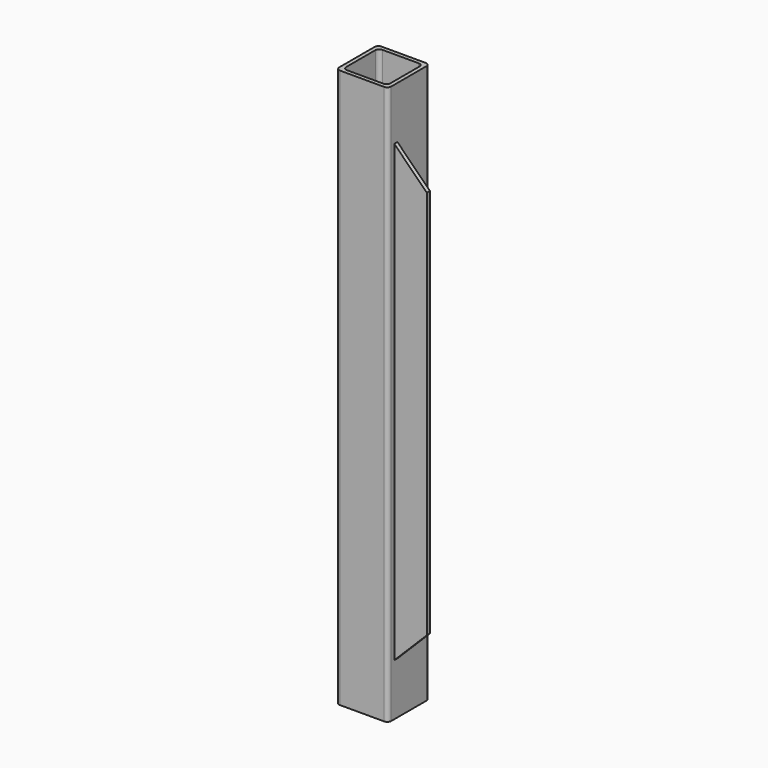
from build123d import *

# Parameters (mm, degrees)
F1_DEPTH = 175
F2_W     = 3
F2_H     = 350
F3_DEPTH = 25
F5_DEPTH = 34.001
F7_DEPTH = 40


# Not quite as in the source:
# - a pattern or mirror of a feature is missing from the dataset's text; its kind, count and spacing are read off the source's solid


with BuildPart() as f1:
    # F0 (on Top) → F1 (new body, symmetric)
    with BuildSketch(Plane.XY):
        with BuildLine():
            ThreePointArc((20, 17), (19.1213203436, 19.1213203436), (17, 20))
            Line((17, 20), (-17, 20))
            ThreePointArc((-17, 20), (-19.1213203436, 19.1213203436), (-20, 17))
            Line((-20, 17), (-20, -17))
            ThreePointArc((-20, -17), (-19.1213203436, -19.1213203436), (-17, -20))
            Line((-17, -20), (17, -20))
            ThreePointArc((17, -20), (19.1213203436, -19.1213203436), (20, -17))
            Line((20, -17), (20, 17))
        make_face()
        with BuildLine():
            ThreePointArc((14, 17), (16.1213203436, 16.1213203436), (17, 14))
            Line((17, 14), (17, -14))
            ThreePointArc((17, -14), (16.1213203436, -16.1213203436), (14, -17))
            Line((14, -17), (-14, -17))
            ThreePointArc((-14, -17), (-16.1213203436, -16.1213203436), (-17, -14))
            Line((-17, -14), (-17, 14))
            ThreePointArc((-17, 14), (-16.1213203436, 16.1213203436), (-14, 17))
            Line((-14, 17), (14, 17))
        make_face(mode=Mode.SUBTRACT)
    extrude(amount=F1_DEPTH, both=True)

    # F2 (on face) → F3 (join)
    with BuildSketch(Plane.YZ.offset(20)):
        with Locations((-12.5, 0)):
            Rectangle(F2_W, F2_H)
    extrude(amount=F3_DEPTH)

    # F4 (on face) → F5 (cut, through all)
    with BuildSketch(Plane.XZ.offset(14)):
        Polygon((45, 175), (20, 175), (45, 150), align=None)
    f5 = extrude(amount=-F5_DEPTH, mode=Mode.SUBTRACT)

    # F5_copies: F5 across plane
    add(f5.mirror(Plane(origin=(0, 0, 0), x_dir=(-1, 0, 0), z_dir=(0, 0, -1))), mode=Mode.SUBTRACT)

    # F6 (on face) → F7 (join)
    with BuildSketch(Plane.XY.offset(175)):
        with BuildLine():
            Line((-20, 17), (-20, -17))
            ThreePointArc((-20, -17), (-19.1213203436, -19.1213203436), (-17, -20))
            Line((-17, -20), (17, -20))
            ThreePointArc((17, -20), (19.1213203436, -19.1213203436), (20, -17))
            Line((20, -17), (20, -14))
            Line((20, -14), (20, -11))
            Line((20, -11), (20, 17))
            ThreePointArc((20, 17), (19.1213203436, 19.1213203436), (17, 20))
            Line((17, 20), (-17, 20))
            ThreePointArc((-17, 20), (-19.1213203436, 19.1213203436), (-20, 17))
        make_face()
        with BuildLine():
            ThreePointArc((-14, -17), (-16.1213203436, -16.1213203436), (-17, -14))
            Line((-17, -14), (-17, 14))
            ThreePointArc((-17, 14), (-16.1213203436, 16.1213203436), (-14, 17))
            Line((-14, 17), (14, 17))
            ThreePointArc((14, 17), (16.1213203436, 16.1213203436), (17, 14))
            Line((17, 14), (17, -14))
            ThreePointArc((17, -14), (16.1213203436, -16.1213203436), (14, -17))
            Line((14, -17), (-14, -17))
        make_face(mode=Mode.SUBTRACT)
    f7 = extrude(amount=F7_DEPTH)

    # F7_copies: F7 across plane
    add(f7.mirror(Plane(origin=(0, 0, 0), x_dir=(-1, 0, 0), z_dir=(0, 0, -1))))


solid = f1.part
